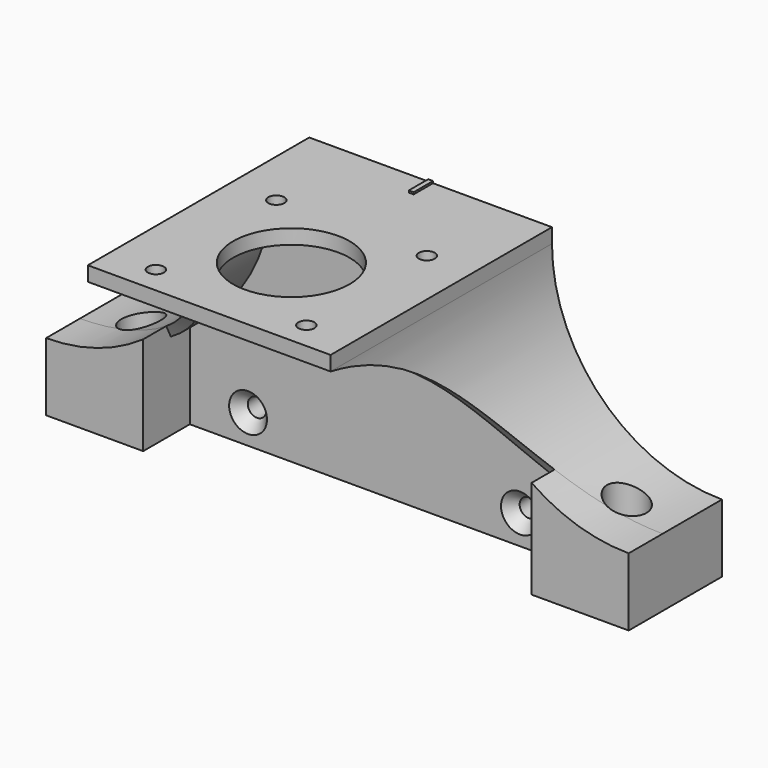
from build123d import *

# Parameters (mm, degrees)
F0_W           = 50
F0_H           = 3
F1_DEPTH       = 12
F3_DEPTH       = 45
F5_DEPTH       = 120.001
F6_R           = 12
F6_R_2         = 1.65
F7_DEPTH       = 25
F9_D           = 3.7973
F9_CSINK_D     = 7.7978
F9_CSINK_ANGLE = 82
F10_W          = 1
F10_H          = 5
F11_DEPTH      = 0.4
F13_END_RADIUS = 35
F13_REACH      = 75.7248075794
F14_END_RADIUS = 35
F14_REACH      = 75.7248075794
F15_DEPTH      = 25


with BuildPart() as f1:
    # F0 (on Front) → F1 (new body)
    with BuildSketch(Plane.XZ):
        with BuildLine():
            Line((22.8227958083, 19.723181963), (-27.1772041917, 19.723181963))
            ThreePointArc((-27.1772041917, 19.723181963), (-37.4284668502, -5.0255553786), (-62.1772041917, -15.276818037))
            Line((-62.1772041917, -15.276818037), (-62.1772041917, -29.276818037))
            Line((-62.1772041917, -29.276818037), (57.8227958083, -29.276818037))
            Line((57.8227958083, -29.276818037), (57.8227958083, -15.276818037))
            ThreePointArc((57.8227958083, -15.276818037), (33.0740584668, -5.0255553786), (22.8227958083, 19.723181963))
        make_face()
        with Locations((-2.1772041917, 21.223181963)):
            Rectangle(F0_W, F0_H)
    extrude(amount=F1_DEPTH)

    # F2 (on face) → F3 (join)
    with BuildSketch(Plane.XZ.offset(12)):
        with BuildLine():
            Line((-25.1772041917, 19.723181963), (-27.1772041917, 19.723181963))
            ThreePointArc((-27.1772041917, 19.723181963), (-37.4284668502, -5.0255553786), (-62.1772041917, -15.276818037))
            Line((-62.1772041917, -15.276818037), (-62.1772041917, -29.276818037))
            Line((-62.1772041917, -29.276818037), (-60.1772041917, -29.276818037))
            Line((-60.1772041917, -29.276818037), (-60.1772041917, -17.2227244409))
            ThreePointArc((-60.1772041917, -17.2227244409), (-35.3164521546, -5.722839337), (-25.1772041917, 19.723181963))
        make_face()
        Polygon((-27.1772041917, 22.723181963), (-27.1772041917, 19.723181963), (-25.1772041917, 19.723181963), (20.8227958083, 19.723181963), (22.8227958083, 19.723181963), (22.8227958083, 22.723181963), align=None)
        with BuildLine():
            Line((22.8227958083, 19.723181963), (20.8227958083, 19.723181963))
            ThreePointArc((20.8227958083, 19.723181963), (30.9620437712, -5.722839337), (55.8227958083, -17.2227244409))
            Line((55.8227958083, -17.2227244409), (55.8227958083, -29.276818037))
            Line((55.8227958083, -29.276818037), (57.8227958083, -29.276818037))
            Line((57.8227958083, -29.276818037), (57.8227958083, -15.276818037))
            ThreePointArc((57.8227958083, -15.276818037), (33.0740584668, -5.0255553786), (22.8227958083, 19.723181963))
        make_face()
    extrude(amount=F3_DEPTH)

    # F4 (on face) → F5 (cut, through all)
    with BuildSketch(Plane(origin=(-62.1772041917, 0, 0), x_dir=(0, -1, 0), z_dir=(-1, 0, 0))):
        with BuildLine():
            Line((57, -15.276818037), (57, 19.723181963))
            ThreePointArc((57, 19.723181963), (26.3280584166, 2.7280262742), (12, -29.276818037))
            Line((12, -29.276818037), (57, -29.276818037))
            Line((57, -29.276818037), (57, -15.276818037))
        make_face()
    extrude(amount=-F5_DEPTH, mode=Mode.SUBTRACT)

    # F6 (on face) → F7 (cut)
    with BuildSketch(Plane.XY.offset(22.723181963)):
        with Locations((-2.1772041917, -35.85)):
            Circle(F6_R)
        with Locations((-17.6772041917, -51.35)):
            Circle(F6_R_2)
        with Locations((-17.6772041917, -20.35)):
            Circle(F6_R_2)
        with Locations((13.3227958083, -51.35)):
            Circle(F6_R_2)
        with Locations((13.3227958083, -20.35)):
            Circle(F6_R_2)
    extrude(amount=-F7_DEPTH, mode=Mode.SUBTRACT)

    # F9 (through all)
    with Locations(Plane.XZ.offset(12)):
        with Locations((-30.1772041917, -23.2497712389), (25.8227958083, -23.2497712389)):
            CounterSinkHole(F9_D / 2, F9_CSINK_D / 2, counter_sink_angle=F9_CSINK_ANGLE)

    # F10 (on face) → F11 (join)
    with BuildSketch(Plane.XY.offset(22.723181963)):
        with Locations((-2.1772041917, -2.5)):
            Rectangle(F10_W, F10_H)
    extrude(amount=F11_DEPTH)

    f13_end = (Plane(origin=(-62.1772041917, -28.5, 19.723181963), x_dir=(0, 0, 1), z_dir=(0, 1, 0)) * Cylinder(F13_END_RADIUS, 437.0700631752, mode=Mode.PRIVATE)).faces().sort_by_distance((-37.4284668502, -0.7549172174, -5.0255553786))[0]
    # F12 (on face) → F13 (join, up to the whole of a round face its end follows)
    with BuildSketch(Plane(origin=(0, 0, -29.276818037), x_dir=(1, 0, 0), z_dir=(0, 0, -1))):
        with BuildLine():
            Line((-62.1772041917, 24), (-62.1772041917, 12))
            Line((-62.1772041917, 12), (-60.1772041917, 12))
            Line((-60.1772041917, 12), (-56.2272041917, 12))
            ThreePointArc((-56.2272041917, 12), (-52.1772041917, 16.05), (-48.1272041917, 12))
            Line((-48.1272041917, 12), (-42.1772041917, 12))
            Line((-42.1772041917, 12), (-42.1772041917, 24))
            Line((-42.1772041917, 24), (-62.1772041917, 24))
        make_face()
        with BuildLine():
            Line((-56.2272041917, 12), (-48.1272041917, 12))
            ThreePointArc((-48.1272041917, 12), (-52.1772041917, 16.05), (-56.2272041917, 12))
        make_face()
    f13_long = extrude(amount=-F13_REACH, mode=Mode.PRIVATE)
    add(split(f13_long, bisect_by=f13_end, keep=Keep.TOP, mode=Mode.PRIVATE))

    f14_end = (Plane(origin=(57.8227958083, -28.5, 19.723181963), x_dir=(0, 0, 1), z_dir=(0, 1, 0)) * Cylinder(F14_END_RADIUS, 437.0700631752, mode=Mode.PRIVATE)).faces().sort_by_distance((33.0740584668, -0.7549172174, -5.0255553786))[0]
    # F12 (on face) → F14 (join, up to the whole of a round face its end follows)
    with BuildSketch(Plane(origin=(0, 0, -29.276818037), x_dir=(1, 0, 0), z_dir=(0, 0, -1))):
        with BuildLine():
            Line((37.8227958083, 24), (37.8227958083, 12))
            Line((37.8227958083, 12), (43.7727958083, 12))
            ThreePointArc((43.7727958083, 12), (47.8227958083, 16.05), (51.8727958083, 12))
            Line((51.8727958083, 12), (55.8227958083, 12))
            Line((55.8227958083, 12), (57.8227958083, 12))
            Line((57.8227958083, 12), (57.8227958083, 24))
            Line((57.8227958083, 24), (37.8227958083, 24))
        make_face()
        with BuildLine():
            Line((51.8727958083, 12), (43.7727958083, 12))
            ThreePointArc((43.7727958083, 12), (47.8227958083, 7.95), (51.8727958083, 12))
        make_face()
    f14_long = extrude(amount=-F14_REACH, mode=Mode.PRIVATE)
    add(split(f14_long, bisect_by=f14_end, keep=Keep.TOP, mode=Mode.PRIVATE))

    # F12 (on face) → F15 (cut)
    with BuildSketch(Plane(origin=(0, 0, -29.276818037), x_dir=(1, 0, 0), z_dir=(0, 0, -1))):
        with BuildLine():
            Line((-56.2272041917, 12), (-48.1272041917, 12))
            ThreePointArc((-48.1272041917, 12), (-52.1772041917, 16.05), (-56.2272041917, 12))
        make_face()
        with BuildLine():
            ThreePointArc((-56.2272041917, 12), (-52.1772041917, 7.95), (-48.1272041917, 12))
            Line((-48.1272041917, 12), (-56.2272041917, 12))
        make_face()
        with BuildLine():
            Line((51.8727958083, 12), (43.7727958083, 12))
            ThreePointArc((43.7727958083, 12), (47.8227958083, 7.95), (51.8727958083, 12))
        make_face()
        with BuildLine():
            ThreePointArc((51.8727958083, 12), (47.8227958083, 16.05), (43.7727958083, 12))
            Line((43.7727958083, 12), (51.8727958083, 12))
        make_face()
    extrude(amount=-F15_DEPTH, mode=Mode.SUBTRACT)


solid = f1.part
